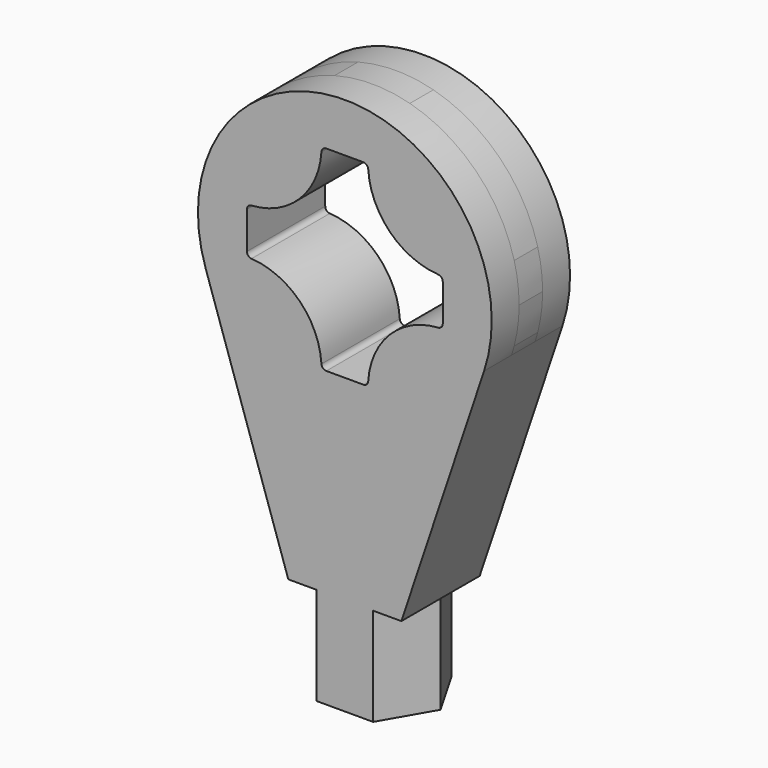
from build123d import *

# Parameters (mm, degrees)
F1_DEPTH   = 3
F5_DEPTH   = 10
F7_DEPTH   = 3
F1_FACE1_R = 15
F8_DEPTH   = 3.5
F1_FACE_R  = 15
F9_DEPTH   = 3.5
F11_R      = 0.5


with BuildPart() as f1:
    # F0 (on Front) → F1 (new body)
    with BuildSketch(Plane.XZ):
        with BuildLine():
            Line((-10, -2.375), (-10, 2.375))
            ThreePointArc((-10, 2.375), (-12.3664158462, 2.7515035323), (-14.4991362367, 3.8438325133))
            ThreePointArc((-14.4991362367, 3.8438325133), (-15, 0), (-14.4991362367, -3.8438325133))
            ThreePointArc((-14.4991362367, -3.8438325133), (-12.3664158462, -2.7515035323), (-10, -2.375))
        make_face()
        with BuildLine():
            Line((-10, 10), (-2.375, 10))
            ThreePointArc((-2.375, 10), (-2.7515035323, 12.3664158462), (-3.8438325133, 14.4991362367))
            ThreePointArc((-3.8438325133, 14.4991362367), (-10.6066017178, 10.6066017178), (-14.4991362367, 3.8438325133))
            ThreePointArc((-14.4991362367, 3.8438325133), (-12.3664158462, 2.7515035323), (-10, 2.375))
            Line((-10, 2.375), (-10, 10))
        make_face()
        with BuildLine():
            ThreePointArc((-10, 2.375), (-4.6083107935, 4.6083107935), (-2.375, 10))
            Line((-2.375, 10), (-10, 10))
            Line((-10, 10), (-10, 2.375))
        make_face()
        with BuildLine():
            Line((-2.375, 10), (2.375, 10))
            ThreePointArc((2.375, 10), (2.7515035323, 12.3664158462), (3.8438325133, 14.4991362367))
            ThreePointArc((3.8438325133, 14.4991362367), (0, 15), (-3.8438325133, 14.4991362367))
            ThreePointArc((-3.8438325133, 14.4991362367), (-2.7515035323, 12.3664158462), (-2.375, 10))
        make_face()
        with BuildLine():
            Line((2.375, 10), (10, 10))
            Line((10, 10), (10, 2.375))
            ThreePointArc((10, 2.375), (12.3664158462, 2.7515035323), (14.4991362367, 3.8438325133))
            ThreePointArc((14.4991362367, 3.8438325133), (10.6066017178, 10.6066017178), (3.8438325133, 14.4991362367))
            ThreePointArc((3.8438325133, 14.4991362367), (2.7515035323, 12.3664158462), (2.375, 10))
        make_face()
        with BuildLine():
            ThreePointArc((14.4991362367, 3.8438325133), (12.3664158462, 2.7515035323), (10, 2.375))
            Line((10, 2.375), (10, -2.375))
            ThreePointArc((10, -2.375), (12.3664158462, -2.7515035323), (14.4991362367, -3.8438325133))
            ThreePointArc((14.4991362367, -3.8438325133), (14.8742570159, -1.9381636218), (15, 0))
            ThreePointArc((15, 0), (14.8742570159, 1.9381636218), (14.4991362367, 3.8438325133))
        make_face()
        with BuildLine():
            ThreePointArc((14.4991362367, -3.8438325133), (12.3664158462, -2.7515035323), (10, -2.375))
            Line((10, -2.375), (10, -10))
            Line((10, -10), (2.375, -10))
            ThreePointArc((2.375, -10), (2.7515035323, -12.3664158462), (3.8438325133, -14.4991362367))
            ThreePointArc((3.8438325133, -14.4991362367), (10.6066017178, -10.6066017178), (14.4991362367, -3.8438325133))
        make_face()
        with BuildLine():
            ThreePointArc((3.8438325133, -14.4991362367), (2.7515035323, -12.3664158462), (2.375, -10))
            Line((2.375, -10), (-2.375, -10))
            ThreePointArc((-2.375, -10), (-2.7515035323, -12.3664158462), (-3.8438325133, -14.4991362367))
            ThreePointArc((-3.8438325133, -14.4991362367), (0, -15), (3.8438325133, -14.4991362367))
        make_face()
        with BuildLine():
            Line((-10, -10), (-10, -2.375))
            ThreePointArc((-10, -2.375), (-12.3664158462, -2.7515035323), (-14.4991362367, -3.8438325133))
            ThreePointArc((-14.4991362367, -3.8438325133), (-10.6066017178, -10.6066017178), (-3.8438325133, -14.4991362367))
            ThreePointArc((-3.8438325133, -14.4991362367), (-2.7515035323, -12.3664158462), (-2.375, -10))
            Line((-2.375, -10), (-10, -10))
        make_face()
        with BuildLine():
            ThreePointArc((-2.375, -10), (-4.6083107935, -4.6083107935), (-10, -2.375))
            Line((-10, -2.375), (-10, -10))
            Line((-10, -10), (-2.375, -10))
        make_face()
        with BuildLine():
            Line((10, -10), (10, -2.375))
            ThreePointArc((10, -2.375), (4.6083107935, -4.6083107935), (2.375, -10))
            Line((2.375, -10), (10, -10))
        make_face()
        with BuildLine():
            Line((10, 2.375), (10, 10))
            Line((10, 10), (2.375, 10))
            ThreePointArc((2.375, 10), (4.6083107935, 4.6083107935), (10, 2.375))
        make_face()
    extrude(amount=F1_DEPTH)


with BuildPart() as f5:
    # F4 (on offset) → F5 (new body)
    with BuildSketch(Plane.XY.offset(-40)):
        Polygon((2.8867513459, 3.5), (-2.8867513459, 3.5), (-5.7735026919, -1.5), (-2.8867513459, -6.5), (2.8867513459, -6.5), (5.7735026919, -1.5), align=None)
    extrude(amount=F5_DEPTH)


with BuildPart() as f7:
    # F6 (on face) → F7 (new body, through all)
    with BuildSketch(Plane(origin=(0, 0, 0), x_dir=(-1, 0, 0), z_dir=(0, 1, 0))):
        with BuildLine():
            ThreePointArc((14.2238332207, -4.7626220204), (0, -15), (-14.2238332207, -4.7626220204))
            Line((-14.2238332207, -4.7626220204), (-5.7735026919, -30))
            Line((-5.7735026919, -30), (5.7735026919, -30))
            Line((5.7735026919, -30), (14.2238332207, -4.7626220204))
        make_face()
    extrude(amount=-F7_DEPTH)


with BuildPart() as f8:
    # F7_face (on face) + F1_face1 (on face) → F8 (new body, through all)
    with BuildSketch(Plane(origin=(0, 0, -20.4204827201), x_dir=(-1, 0, 0), z_dir=(0, 1, 0))):
        with BuildLine():
            ThreePointArc((14.2238332207, 15.6578606997), (0, 5.4204827201), (-14.2238332207, 15.6578606997))
            Line((-14.2238332207, 15.6578606997), (-5.7735026919, -9.5795172799))
            Line((-5.7735026919, -9.5795172799), (5.7735026919, -9.5795172799))
            Line((5.7735026919, -9.5795172799), (14.2238332207, 15.6578606997))
        make_face()
    with BuildSketch(Plane(origin=(0, 0, 0), x_dir=(1, 0, 0), z_dir=(0, 1, 0))):
        Circle(F1_FACE1_R)
        with BuildLine():
            ThreePointArc((-2.375, -10), (-4.6083107935, -4.6083107935), (-10, -2.375))
            Line((-10, -2.375), (-10, 2.375))
            ThreePointArc((-10, 2.375), (-4.6083107935, 4.6083107935), (-2.375, 10))
            Line((-2.375, 10), (2.375, 10))
            ThreePointArc((2.375, 10), (4.6083107935, 4.6083107935), (10, 2.375))
            Line((10, 2.375), (10, -2.375))
            ThreePointArc((10, -2.375), (4.6083107935, -4.6083107935), (2.375, -10))
            Line((2.375, -10), (-2.375, -10))
        make_face(mode=Mode.SUBTRACT)
    extrude(amount=F8_DEPTH)


with BuildPart() as f9:
    # F1_face (on face) + F7_face1 (on face) → F9 (new body, through all)
    with BuildSketch(Plane.XZ.offset(3)):
        Circle(F1_FACE_R)
        with BuildLine():
            ThreePointArc((-10, 2.375), (-4.6083107935, 4.6083107935), (-2.375, 10))
            Line((-2.375, 10), (2.375, 10))
            ThreePointArc((2.375, 10), (4.6083107935, 4.6083107935), (10, 2.375))
            Line((10, 2.375), (10, -2.375))
            ThreePointArc((10, -2.375), (4.6083107935, -4.6083107935), (2.375, -10))
            Line((2.375, -10), (-2.375, -10))
            ThreePointArc((-2.375, -10), (-4.6083107935, -4.6083107935), (-10, -2.375))
            Line((-10, -2.375), (-10, 2.375))
        make_face(mode=Mode.SUBTRACT)
    with BuildSketch(Plane(origin=(0, -3, -20.4204827201), x_dir=(-1, 0, 0), z_dir=(0, -1, 0))):
        with BuildLine():
            ThreePointArc((-14.2238332207, -15.6578606997), (0, -5.4204827201), (14.2238332207, -15.6578606997))
            Line((14.2238332207, -15.6578606997), (5.7735026919, 9.5795172799))
            Line((5.7735026919, 9.5795172799), (-5.7735026919, 9.5795172799))
            Line((-5.7735026919, 9.5795172799), (-14.2238332207, -15.6578606997))
        make_face()
    extrude(amount=F9_DEPTH)


with BuildPart() as f5_1:
    add(f5.part)

    # F10: union F8, F7, F9, F1
    add(f8.part)
    add(f7.part)
    add(f9.part)
    add(f1.part)

    # F11
    f11_edges = [f5_1.edges().sort_by_distance(p)[0] for p in [
        (10, -1.5, -2.375),
        (10, -1.5, 2.375),
        (2.375, -1.5, -10),
        (-2.375, -1.5, -10),
        (-10, -1.5, -2.375),
        (-10, -1.5, 2.375),
        (-2.375, -1.5, 10),
        (2.375, -1.5, 10),
    ]]
    fillet(f11_edges, radius=F11_R)


solid = f5_1.part
